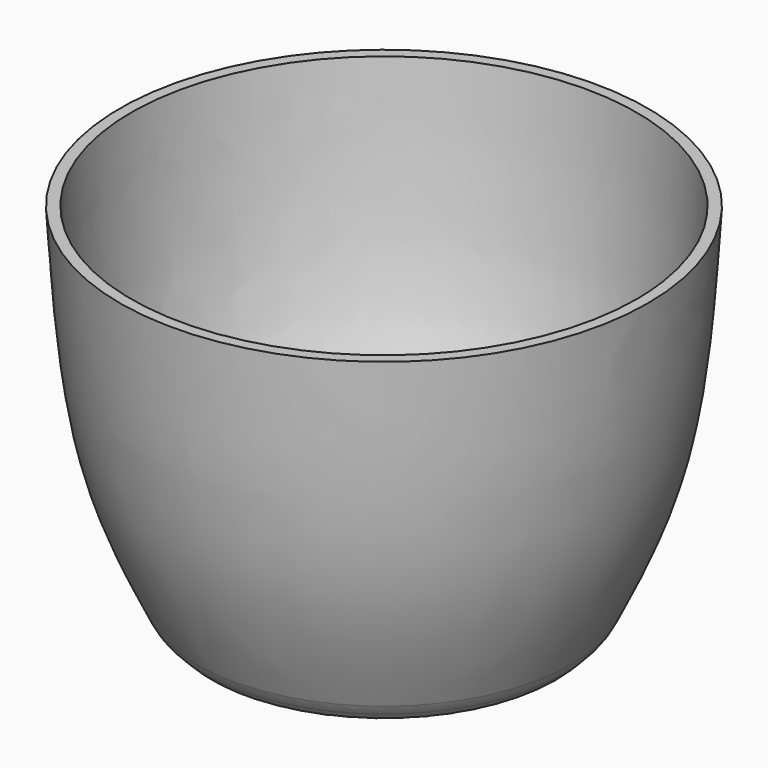
from build123d import *

# Parameters (mm, degrees)
F2_T = -20.32


with BuildPart() as f1:
    # F0 (on Front) → F1 (revolve)
    with BuildSketch(Plane.XZ):
        with BuildLine():
            Line((0, 635), (0, 0))
            Line((0, 0), (247.2740947085, 0))
            ThreePointArc((247.2740947085, 0), (253.2179086611, -1.4767617999), (257.779423812, -5.5636101265))
            Line((257.779423812, -5.5636101265), (267.4750858754, -19.8363898735))
            ThreePointArc((267.4750858754, -19.8363898735), (272.0366010263, -23.9232382001), (277.980414979, -25.4))
            Line((277.980414979, -25.4), (304.0896017916, -25.4))
            ThreePointArc((304.0896017916, -25.4), (308.9531470731, -24.4318339272), (313.0751617192, -21.6749491802))
            Line((313.0751617192, -21.6749491802), (325.8108005635, -8.9242534656))
            ThreePointArc((325.8108005635, -8.9242534656), (333.9006905197, 0.6305542274), (340.3168473718, 11.3810705313))
            add(Edge.make_bspline(
                [(340.3168473718, 11.3810705313), (376.7943098118, 85.7830117652), (455.8228488247, 255.712567795), (471.5220391728, 499.1467710715), (479.8279702663, 635)],
                knots=[0.0220814037, 0.0220814037, 0.0220814037, 0.0220814037, 0.4549677561, 1, 1, 1, 1], degree=3))
            Line((479.8279702663, 635), (0, 635))
        make_face()
    revolve(axis=Axis((0, 0, 317.5), (0, 0, 1)))

    # F2
    f2_openings = [f1.faces().sort_by_distance(p)[0] for p in [
        (0, 0, 635),
    ]]
    offset(amount=F2_T, openings=f2_openings)


solid = f1.part
